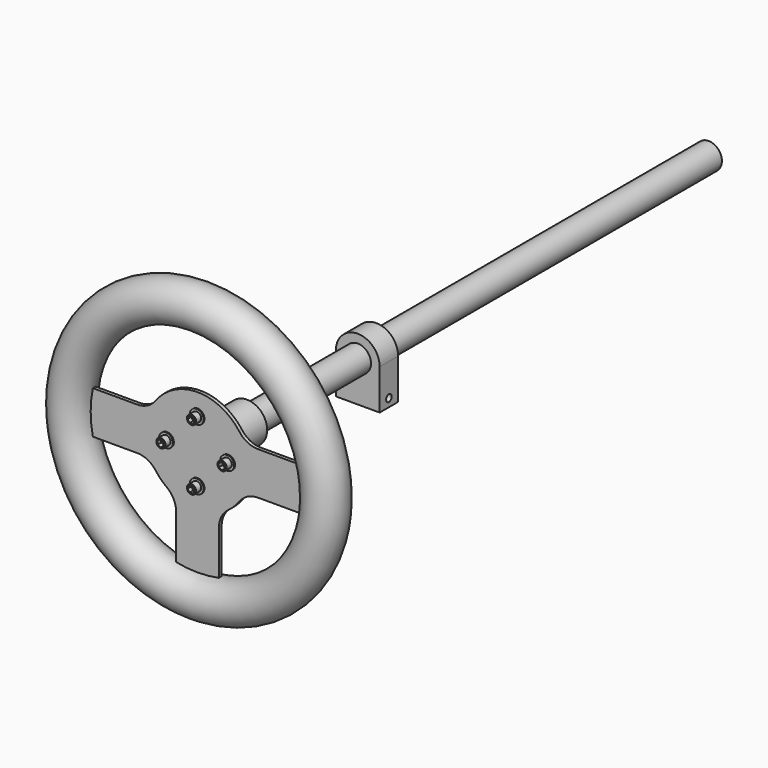
from build123d import *

# Parameters (mm, degrees)
F0_R             = 11.5
F1_DEPTH         = 500
F2_R             = 17.5
F3_DEPTH         = 52
F5_R             = 17.5
F8_DEPTH         = 1.5
F10_R            = 11.5
F11_DEPTH        = 20
F12_R            = 3
F13_DEPTH        = 25
F14_R            = 6
F15_DEPTH        = 1
F15_COPIES_COUNT = 4
F16_R            = 4
F17_DEPTH        = 6
F17_COPIES_COUNT = 4
F19_DEPTH        = 4
F19_COPIES_COUNT = 4
F20_SIZE         = 0.5


# Not quite as in the source:
# - a pattern or mirror of a feature is missing from the dataset's text; its kind, count and spacing are read off the source's solid


with BuildPart() as f1:
    # F0 (on Front) → F1 (new body)
    with BuildSketch(Plane.XZ):
        Circle(F0_R)
    extrude(amount=F1_DEPTH)

    # F2 (on face) → F3 (join)
    with BuildSketch(Plane.XZ.offset(500)):
        Circle(F2_R)
    extrude(amount=F3_DEPTH)



with BuildPart() as f6:
    # F5 (on Right) → F6 (revolve)
    with BuildSketch(Plane.YZ):
        with Locations((-552, 110)):
            Circle(F5_R)
    revolve(axis=Axis((0, -586.2022111416, 0), (0, -1, 0)))


with BuildPart() as f1_1:
    add(f1.part)

    add(f6.part)  # F8 merges F6
    # F7 (on face) → F8 (join, symmetric)
    with BuildSketch(Plane.XZ.offset(552)):
        with BuildLine():
            ThreePointArc((-52.3712707503, -18.5), (-43.3414057713, -20.6545092961), (-36.2570335964, -26.6538461538))
            ThreePointArc((-36.2570335964, -26.6538461538), (-31.8198051534, -31.8198051534), (-26.6538461538, -36.2570335964))
            ThreePointArc((-26.6538461538, -36.2570335964), (-20.6545092961, -43.3414057713), (-18.5, -52.3712707503))
            Line((-18.5, -52.3712707503), (-18.5, -101.6479799574))
            ThreePointArc((-18.5, -101.6479799574), (0, -103.317771121), (18.5, -101.6479799574))
            Line((18.5, -101.6479799574), (18.5, -52.3712707503))
            ThreePointArc((18.5, -52.3712707503), (20.6545092961, -43.3414057713), (26.6538461538, -36.2570335964))
            ThreePointArc((26.6538461538, -36.2570335964), (31.8198051534, -31.8198051534), (36.2570335964, -26.6538461538))
            ThreePointArc((36.2570335964, -26.6538461538), (43.3414057713, -20.6545092961), (52.3712707503, -18.5))
            Line((52.3712707503, -18.5), (101.6479799574, -18.5))
            ThreePointArc((101.6479799574, -18.5), (103.317771121, 0), (101.6479799574, 18.5))
            Line((101.6479799574, 18.5), (52.3712707503, 18.5))
            ThreePointArc((52.3712707503, 18.5), (43.3414057713, 20.6545092961), (36.2570335964, 26.6538461538))
            ThreePointArc((36.2570335964, 26.6538461538), (0, 45), (-36.2570335964, 26.6538461538))
            ThreePointArc((-36.2570335964, 26.6538461538), (-43.3414057713, 20.6545092961), (-52.3712707503, 18.5))
            Line((-52.3712707503, 18.5), (-101.6479799574, 18.5))
            ThreePointArc((-101.6479799574, 18.5), (-103.317771121, 0), (-101.6479799574, -18.5))
            Line((-101.6479799574, -18.5), (-52.3712707503, -18.5))
        make_face()
    extrude(amount=F8_DEPTH, both=True)

    # F10 (on offset) → F11 (join)
    with BuildSketch(Plane(origin=(0, -380, 0), x_dir=(-1, 0, 0), z_dir=(0, 1, 0))):
        with BuildLine():
            Line((19, -35), (19, 0))
            ThreePointArc((19, 0), (0, 19), (-19, 0))
            Line((-19, 0), (-19, -35))
            Line((-19, -35), (19, -35))
        make_face()
        Circle(F10_R, mode=Mode.SUBTRACT)
    extrude(amount=F11_DEPTH)

    # F12 (on face) → F13 (cut)
    with BuildSketch(Plane.YZ.offset(19)):
        with Locations((-370, -28)):
            Circle(F12_R)
    extrude(amount=-F13_DEPTH, mode=Mode.SUBTRACT)

    # F14 (on face) → F15 (join)
    with BuildSketch(Plane.XZ.offset(553.5)):
        with Locations((0, 26.5213046223)):
            Circle(F14_R)
    f15 = extrude(amount=F15_DEPTH)

    # F15_copies: F15 ×4 about axis
    f15_copies_axis = Axis((0, 0, 0), (0, 1, 0))
    for i in range(1, F15_COPIES_COUNT):
        add(f15.rotate(f15_copies_axis, i * 360 / F15_COPIES_COUNT))

    # F16 (on face) → F17 (join)
    with BuildSketch(Plane.XZ.offset(554.5)):
        with Locations((0, 26.5213046223)):
            Circle(F16_R)
    f17 = extrude(amount=F17_DEPTH)

    # F17_copies: F17 ×4 about axis
    f17_copies_axis = Axis((0, 0, 0), (0, 1, 0))
    for i in range(1, F17_COPIES_COUNT):
        add(f17.rotate(f17_copies_axis, i * 360 / F17_COPIES_COUNT))

    # F18 (on face) → F19 (cut)
    with BuildSketch(Plane.XZ.offset(560.5)):
        Polygon((2.9804941814, 26.7480426348), (1.2938862119, 29.2158573055), (-1.6866079695, 28.989119293), (-2.9804941814, 26.2945666098), (-1.2938862119, 23.8267519391), (1.6866079695, 24.0534899516), align=None)
    f19 = extrude(amount=-F19_DEPTH, mode=Mode.SUBTRACT)

    # F19_copies: F19 ×4 about axis
    f19_copies_axis = Axis((0, 0, 0), (0, 1, 0))
    for i in range(1, F19_COPIES_COUNT):
        add(f19.rotate(f19_copies_axis, i * 360 / F19_COPIES_COUNT), mode=Mode.SUBTRACT)

    # F20
    f20_edges = [f1_1.edges().sort_by_distance(p)[0] for p in [
        (-4, -560.5, 26.521305),
        (-26.521305, -560.5, -4),
        (4, -560.5, -26.521305),
        (26.521305, -560.5, 4),
    ]]
    chamfer(f20_edges, length=F20_SIZE)


solid = f1_1.part
